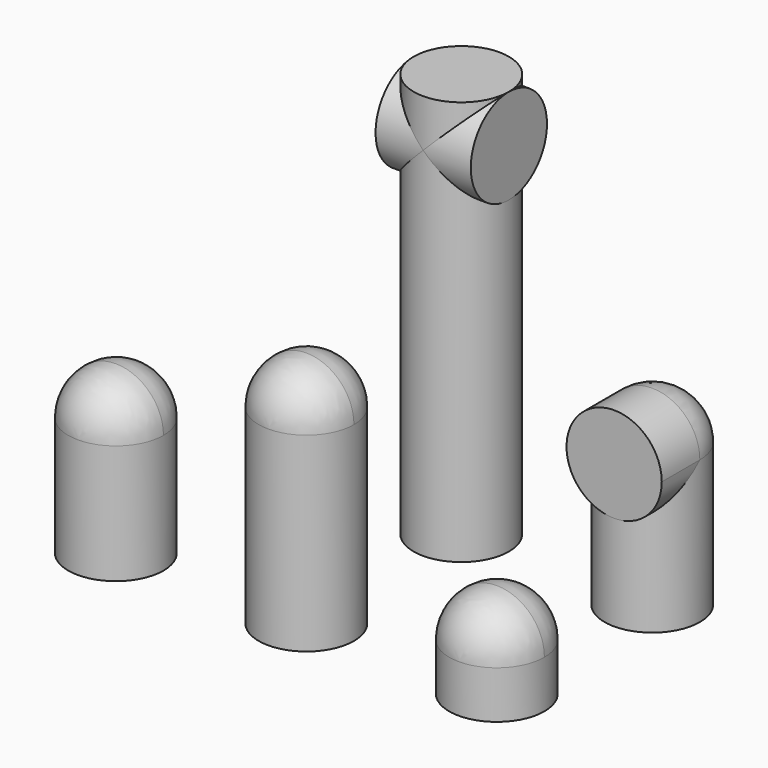
from build123d import *
from build123d import SkipClean  # not in build123d's __all__

# Parameters (mm, degrees)
F0_R          = 10
F1_DEPTH      = 85
F2_R          = 10
F3_DEPTH      = 10
F3_DEPTH_BACK = 10
F4_R          = 10
F5_DEPTH      = 30
F6_R          = 10
F7_DEPTH      = 10
F9_ANGLE      = 90
F10_R         = 10
F11_DEPTH     = 40
F12_DEPTH     = 25
F13_DEPTH     = 10


with BuildPart() as f1:
    # F0 (on Top) → F1 (new body)
    with BuildSketch(Plane.XY):
        Circle(F0_R)
    extrude(amount=F1_DEPTH)

    # F2 (on Right) → F3 (join, two sides)
    with BuildSketch(Plane.YZ) as f3_sk:
        with Locations((0, 75)):
            Circle(F2_R)
    extrude(amount=F3_DEPTH)
    extrude(f3_sk.sketch, amount=-F3_DEPTH_BACK)


with BuildPart() as f5:
    # F4 (on Top) → F5 (new body)
    with BuildSketch(Plane.XY):
        with Locations((40.103476, 0)):
            Circle(F4_R)
    extrude(amount=F5_DEPTH)

    # F6 (on Front) → F7 (join)
    with BuildSketch(Plane.XZ):
        with Locations((40.103476, 30)):
            Circle(F6_R)
    with SkipClean():  # cleaning this boolean's faces spoils the solid; the shape is the same uncleaned
        extrude(amount=F7_DEPTH)

    # F8 (on face) → F9 (revolve)
    with BuildSketch(Plane.XY.offset(30)):
        with BuildLine():
            Line((30.103476, 0), (50.103476, 0))
            ThreePointArc((50.103476, 0), (40.103476, 10), (30.103476, 0))
        make_face()
    with SkipClean():  # cleaning this boolean's faces spoils the solid; the shape is the same uncleaned
        revolve(axis=Axis((40.103476, 0, 30), (1, 0, 0)), revolution_arc=F9_ANGLE)


with BuildPart() as f11:
    # F10 (on Top) → F11 (new body)
    with BuildSketch(Plane.XY):
        with Locations((0, -40.676132)):
            Circle(F10_R)
    extrude(amount=F11_DEPTH)

    # F14 (on face) → F15 (revolve)
    with BuildSketch(Plane.XY.offset(40)):
        with BuildLine():
            ThreePointArc((0, -50.676132), (7.071068, -47.7472), (10, -40.676132))
            ThreePointArc((10, -40.676132), (7.071068, -33.605064), (0, -30.676132))
            Line((0, -30.676132), (0, -50.676132))
        make_face()
    revolve(axis=Axis((0, -40.676132, 40), (0, -1, 0)))


with BuildPart() as f12:
    # F10 (on Top) → F12 (new body)
    with BuildSketch(Plane.XY):
        with Locations((-40, -40.676132)):
            Circle(F10_R)
    extrude(amount=F12_DEPTH)

    # F16 (on face) → F17 (revolve)
    with BuildSketch(Plane.XY.offset(25)):
        with BuildLine():
            ThreePointArc((-40, -50.676132), (-32.928932, -47.7472), (-30, -40.676132))
            ThreePointArc((-30, -40.676132), (-32.928932, -33.605064), (-40, -30.676132))
            Line((-40, -30.676132), (-40, -50.676132))
        make_face()
    revolve(axis=Axis((-40, -40.676132, 25), (0, -1, 0)))


with BuildPart() as f13:
    # F10 (on Top) → F13 (new body)
    with BuildSketch(Plane.XY):
        with Locations((40, -40.676132)):
            Circle(F10_R)
    extrude(amount=F13_DEPTH)

    # F18 (on face) → F19 (revolve)
    with BuildSketch(Plane.XY.offset(10)):
        with BuildLine():
            ThreePointArc((40, -50.676132), (47.071068, -47.7472), (50, -40.676132))
            ThreePointArc((50, -40.676132), (47.071068, -33.605064), (40, -30.676132))
            Line((40, -30.676132), (40, -50.676132))
        make_face()
    revolve(axis=Axis((40, -40.676132, 10), (0, -1, 0)))


solid = Compound([f1.part, f5.part, f11.part, f12.part, f13.part])
